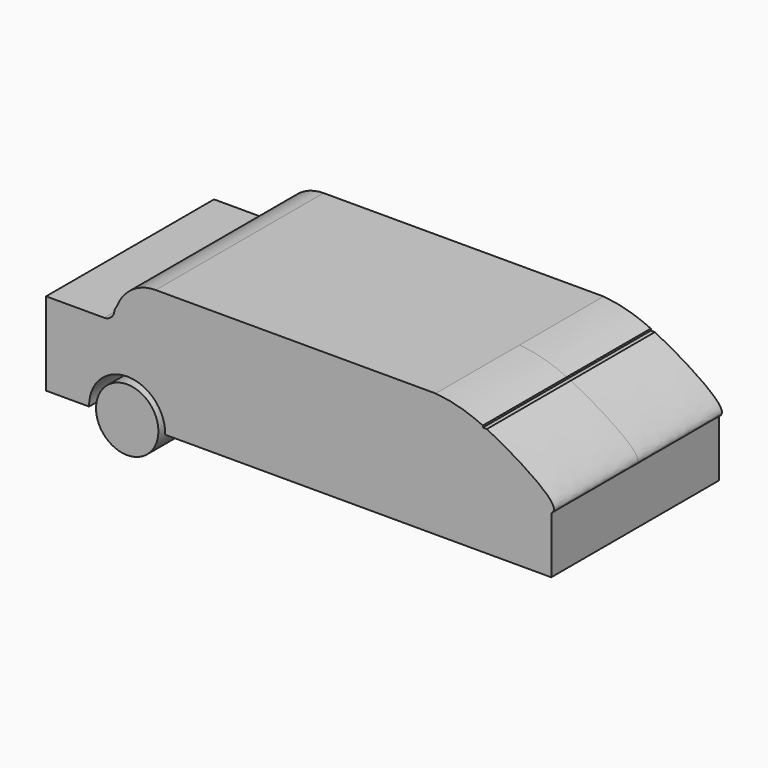
from build123d import *

# Parameters (mm, degrees)
F1_DEPTH  = 51
F3_R      = 18.5060430465
F4_DEPTH  = 127.0010001
F5_R      = 15.1571066155
F6_DEPTH  = 21.1
F10_DEPTH = 10.4
F11_R     = 17.8934815189
F12_DEPTH = 10.5


# Not quite as in the source:
# - the program builds the solid bodies; features that only make, move or delete a surface that nothing else refers to are left out


with BuildPart() as f1:
    # F0 (on Front) → F1 (new body, symmetric)
    with BuildSketch(Plane.XZ):
        with BuildLine():
            Line((-94.4829183817, 20.1827697456), (-122.7041259408, 20.1827697456))
            Line((-122.7041259408, 20.1827697456), (-122.7041259408, -20.1827697456))
            Line((-122.7041259408, -20.1827697456), (122.7041259408, -20.1827697456))
            Line((122.7041259408, -20.1827697456), (122.7041259408, 7.322948426))
            add(Edge.make_bspline(
                [(122.7041259408, 7.322948426), (112.2416987546, 1.2139475694), (-7.7697103098, 23.886095006), (41.1053786314, 39.0712127023), (55.6025840342, 40.1869378984)],
                knots=[0.4436872716, 0.4436872716, 0.4436872716, 0.4436872716, 0.7996841869, 1, 1, 1, 1], degree=3))
            Line((55.6025840342, 40.1869378984), (-69.4829183817, 40.1869378984))
            ThreePointArc((-69.4829183817, 40.1869378984), (-80.7486328998, 36.7121815092), (-88.0997860678, 27.4953055381))
            Line((-88.0997860678, 27.4953055381), (-89.4829183817, 25.1827697456))
            ThreePointArc((-89.4829183817, 25.1827697456), (-90.9473844758, 21.6472358397), (-94.4829183817, 20.1827697456))
        make_face()
        with BuildLine():
            add(Edge.make_bspline(
                [(122.7041259408, 7.322948426), (112.2416987546, 1.2139475694), (-7.7697103098, 23.886095006), (41.1053786314, 39.0712127023), (55.6025840342, 40.1869378984)],
                knots=[0.4436872716, 0.4436872716, 0.4436872716, 0.4436872716, 0.7996841869, 1, 1, 1, 1], degree=3))
            add(Edge.make_bspline(
                [(91.4303071797, 33.0425910673), (95.3213672764, 31.1793724696), (110.5598336265, 22.7600055142), (128.2577602497, 10.5657099904), (122.7041259408, 7.322948426)],
                knots=[0.189121353, 0.189121353, 0.189121353, 0.189121353, 0.2547180537, 0.4436872716, 0.4436872716, 0.4436872716, 0.4436872716], degree=3))
            Line((91.4303071797, 33.0425910673), (89.4829183835, 33.0425910674))
            Line((89.4829183835, 33.0425910674), (89.4829183833, 33.9503373137))
            add(Edge.make_bspline(
                [(66.5373471656, 40.1869378984), (74.7246059451, 39.5132642043), (82.0778170268, 37.3057446954), (89.4829183833, 33.9503373137)],
                knots=[0.0530594435, 0.0530594435, 0.0530594435, 0.0530594435, 0.1781647263, 0.1781647263, 0.1781647263, 0.1781647263], degree=3))
            Line((66.5373471656, 40.1869378984), (55.6025840342, 40.1869378984))
        make_face()
    extrude(amount=F1_DEPTH, both=True)

    # F3 (on offset) → F4 (cut, through all)
    with BuildSketch(Plane.XZ.offset(76)):
        with Locations((-83.3006650209, -19.7968743742)):
            Circle(F3_R)
    extrude(amount=-F4_DEPTH, mode=Mode.SUBTRACT)

    # F9 (on face) → F10 (join, symmetric)
    with BuildSketch(Plane(origin=(0, 51, 0), x_dir=(-1, 0, 0), z_dir=(0, 1, 0))):
        with BuildLine():
            Line((-92.6035834794, -20.1827697456), (-59.6113161798, -20.1827697456))
            ThreePointArc((-59.6113161798, -20.1827697456), (-76.1074498296, -3.6866360958), (-92.6035834794, -20.1827697456))
        make_face()
        with BuildLine():
            ThreePointArc((-92.6035834794, -20.1827697456), (-76.1074498296, -36.6789033954), (-59.6113161798, -20.1827697456))
            Line((-59.6113161798, -20.1827697456), (-92.6035834794, -20.1827697456))
        make_face()
    extrude(amount=F10_DEPTH, both=True)


with BuildPart() as f6:
    # F5 (on face) → F6 (new body)
    with BuildSketch(Plane.XZ.offset(51)):
        with Locations((-83.3006650209, -19.7968743742)):
            Circle(F5_R)
    extrude(amount=-F6_DEPTH)


with BuildPart() as f12:
    # F11 (on face) → F12 (new body, symmetric)
    with BuildSketch(Plane(origin=(0, 51, 0), x_dir=(-1, 0, 0), z_dir=(0, 1, 0))):
        with Locations((83.3006650209, -19.7968743742)):
            Circle(F11_R)
    extrude(amount=F12_DEPTH, both=True)


solid = Compound([f1.part, f6.part, f12.part])
